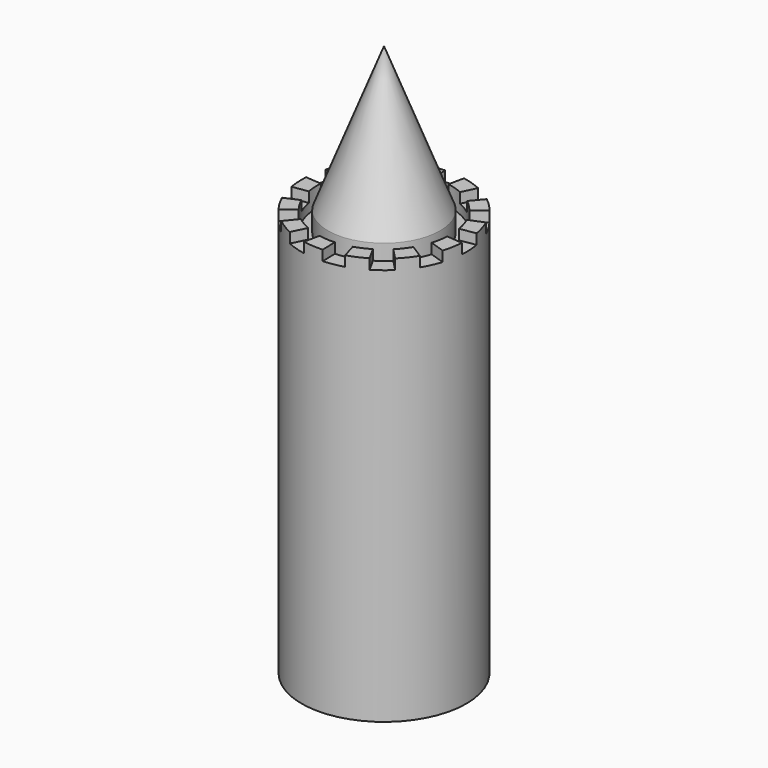
from build123d import *

# Parameters (mm, degrees)
F3_DEPTH        = 1.3
F3_COPIES_COUNT = 13


# Not quite as in the source:
# - a pattern or mirror of a feature is missing from the dataset's text; its kind, count and spacing are read off the source's solid


with BuildPart() as f1:
    # F0 (on Front) → F1 (revolve)
    with BuildSketch(Plane.XZ):
        Polygon((0, 3.4508320969), (0, 0), (10.5, 0), (10.5, 52), (8.5, 52), (8.5, 49.5), (7.1502993815, 49.5), (7.1502993815, 52), (0, 70.4032331705), (0, 44.7733812034), (7.0547335781, 44.7733812034), (7.0547335781, 3.4508320969), align=None)
    revolve(axis=Axis((0, 0, 35.2016165853), (0, 0, 1)))

    # F2 (on face) → F3 (cut)
    with BuildSketch(Plane.XY.offset(52)):
        with BuildLine():
            ThreePointArc((6.5231491988, 8.2279113103), (5.4797365468, 8.9567006971), (4.3558130739, 9.5538940995))
            Line((4.3558130739, 9.5538940995), (3.5032103316, 7.7445153091))
            ThreePointArc((3.5032103316, 7.7445153091), (4.4034584873, 7.2704575751), (5.2406151405, 6.6922307902))
            Line((5.2406151405, 6.6922307902), (6.5231491988, 8.2279113103))
        make_face()
    f3 = extrude(amount=-F3_DEPTH, mode=Mode.SUBTRACT)

    # F3_copies: F3 ×13 about axis
    f3_copies_axis = Axis((0, 0, 0), (0, 0, 1))
    for i in range(1, F3_COPIES_COUNT):
        add(f3.rotate(f3_copies_axis, i * 360 / F3_COPIES_COUNT), mode=Mode.SUBTRACT)


solid = f1.part
